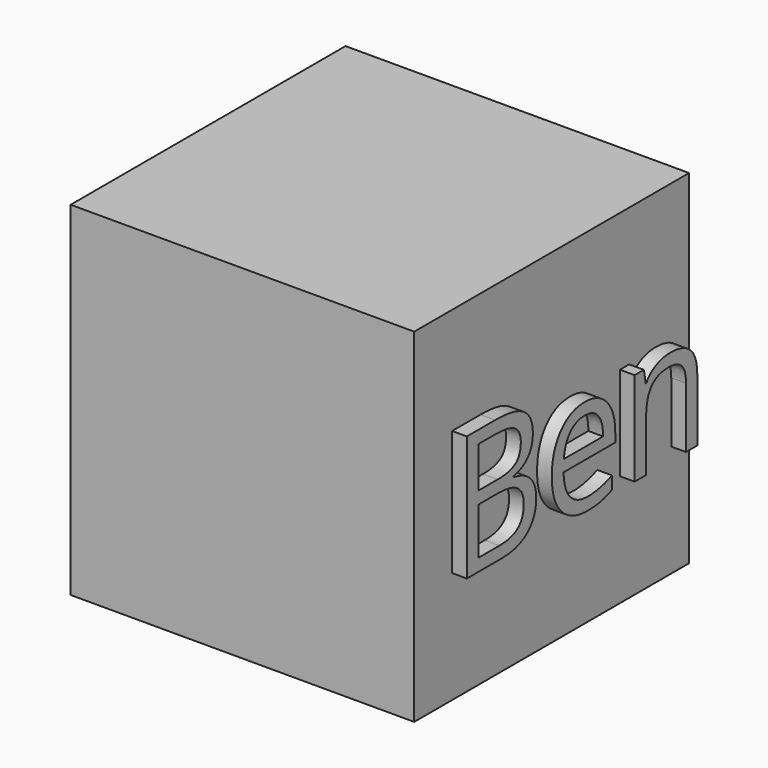
from build123d import *

# Parameters (mm, degrees)
F0_W         = 35
F0_H         = 35
F1_DEPTH     = 35
F2_W         = 29.2401773821
F2_H         = 29.2401773821
F3_DEPTH     = 29.2401773821
F4_TEXT_SIZE = 17.8518329954
F5_DEPTH     = 1.5


# Not quite as in the source:
# - Text() gives the source's letters only with a copy of the font that has no kerning and outlines rounded to 1/6400 em; it was checked with that copy


with BuildPart() as f1:
    # F0 (on Front) → F1 (new body)
    with BuildSketch(Plane.XZ):
        Rectangle(F0_W, F0_H)
    extrude(amount=F1_DEPTH)

    # F2 (on Front) → F3 (cut)
    with BuildSketch(Plane.XZ):
        Rectangle(F2_W, F2_H)
    extrude(amount=F3_DEPTH, mode=Mode.SUBTRACT)

    # F4 (on face) → F5 (join)
    with BuildSketch(Plane.YZ.offset(17.5)):
        with Locations((-31.9259688258, -6.1142556369)):
            Text('Ben', F4_TEXT_SIZE, font='Open Sans', text_align=(TextAlign.LEFT, TextAlign.BOTTOM))
    extrude(amount=F5_DEPTH)


solid = f1.part
